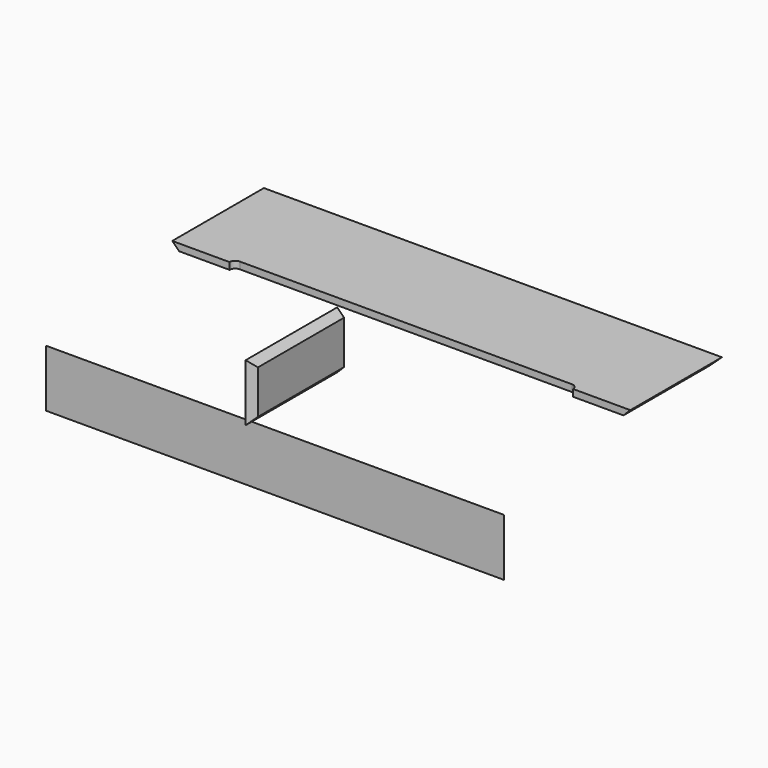
from build123d import *

# Parameters (mm, degrees)
F0_W      = 800
F0_H      = 100
F1_DEPTH  = 12
F2_W      = 200
F2_H      = 100
F3_DEPTH  = 12
F4_SIZE   = 11.99999
F5_SIZE   = 11.99999
F6_SIZE   = 11.99999
F7_W      = 800
F7_H      = 200
F8_DEPTH  = 12
F9_SIZE   = 11.99999
F10_SIZE  = 11.99999
F11_SIZE  = 11.99999
F12_SIZE  = 11.99999
F13_SIZE  = 11.99999
F14_SIZE  = 11.99999
F15_SIZE  = 11.99999
F16_W     = 600
F16_H     = 20
F17_DEPTH = 25
F18_R     = 9.99999
F19_R     = 9.99999


# Not quite as in the source:
# - a fillet or chamfer is up to 0.001 mm smaller than in the source, because OpenCascade refuses the exact size


with BuildPart() as f1:
    # F0 (on Front) → F1 (new body)
    with BuildSketch(Plane.XZ):
        with Locations((-14.225743711, -141.3142682277)):
            Rectangle(F0_W, F0_H)
    extrude(amount=F1_DEPTH)

    # F5 (size 12 in the source; OpenCascade refuses exactly that, so slightly less here)
    f5_edges = [f1.edges().sort_by_distance(p)[0] for p in [
        (-414.225744, 0, -141.314268),
    ]]
    chamfer(f5_edges, length=F5_SIZE)

    # F6 (size 12 in the source; OpenCascade refuses exactly that, so slightly less here)
    f6_edges = [f1.edges().sort_by_distance(p)[0] for p in [
        (385.774256, 0, -141.314268),
    ]]
    chamfer(f6_edges, length=F6_SIZE)

    # F9 (size 12 in the source; OpenCascade refuses exactly that, so slightly less here)
    f9_edges = [f1.edges().sort_by_distance(p)[0] for p in [
        (-14.225744, 0, -91.314268),
    ]]
    chamfer(f9_edges, length=F9_SIZE)

    # F10 (size 12 in the source; OpenCascade refuses exactly that, so slightly less here)
    f10_edges = [f1.edges().sort_by_distance(p)[0] for p in [
        (-14.225744, 0, -191.314268),
    ]]
    chamfer(f10_edges, length=F10_SIZE)


with BuildPart() as f3:
    # F2 (on Right) → F3 (new body)
    with BuildSketch(Plane.YZ):
        with Locations((5.7870447636, 4.5209136379)):
            Rectangle(F2_W, F2_H)
    extrude(amount=F3_DEPTH)

    # F4 (size 12 in the source; OpenCascade refuses exactly that, so slightly less here)
    f4_edges = [f3.edges().sort_by_distance(p)[0] for p in [
        (12, -94.212955, 4.520914),
    ]]
    chamfer(f4_edges, length=F4_SIZE)

    # F14 (size 12 in the source; OpenCascade refuses exactly that, so slightly less here)
    f14_edges = [f3.edges().sort_by_distance(p)[0] for p in [
        (12, 11.78704, 54.520914),
    ]]
    chamfer(f14_edges, length=F14_SIZE)

    # F15 (size 12 in the source; OpenCascade refuses exactly that, so slightly less here)
    f15_edges = [f3.edges().sort_by_distance(p)[0] for p in [
        (12, 11.78704, -45.479086),
    ]]
    chamfer(f15_edges, length=F15_SIZE)


with BuildPart() as f8:
    # F7 (on Top) → F8 (new body)
    with BuildSketch(Plane.XY):
        with Locations((50.7886199192, 282.1810945868)):
            Rectangle(F7_W, F7_H)
    extrude(amount=F8_DEPTH)

    # F11 (size 12 in the source; OpenCascade refuses exactly that, so slightly less here)
    f11_edges = [f8.edges().sort_by_distance(p)[0] for p in [
        (50.78862, 382.181095, 0),
    ]]
    chamfer(f11_edges, length=F11_SIZE)

    # F12 (size 12 in the source; OpenCascade refuses exactly that, so slightly less here)
    f12_edges = [f8.edges().sort_by_distance(p)[0] for p in [
        (-349.21138, 276.1811, 0),
    ]]
    chamfer(f12_edges, length=F12_SIZE)

    # F13 (size 12 in the source; OpenCascade refuses exactly that, so slightly less here)
    f13_edges = [f8.edges().sort_by_distance(p)[0] for p in [
        (450.78862, 276.1811, 0),
    ]]
    chamfer(f13_edges, length=F13_SIZE)

    # F16 (on face) → F17 (cut)
    with BuildSketch(Plane.XY.offset(12)):
        with Locations((50.7886199192, 182.1810945868)):
            Rectangle(F16_W, F16_H)
    extrude(amount=-F17_DEPTH, mode=Mode.SUBTRACT)

    # F18 (radius 10 in the source; OpenCascade refuses exactly that, so slightly less here)
    f18_edges = [f8.edges().sort_by_distance(p)[0] for p in [
        (-249.21138, 192.181095, 6),
    ]]
    fillet(f18_edges, radius=F18_R)

    # F19 (radius 10 in the source; OpenCascade refuses exactly that, so slightly less here)
    f19_edges = [f8.edges().sort_by_distance(p)[0] for p in [
        (350.78862, 192.181095, 6),
    ]]
    fillet(f19_edges, radius=F19_R)


solid = Compound([f1.part, f3.part, f8.part])
